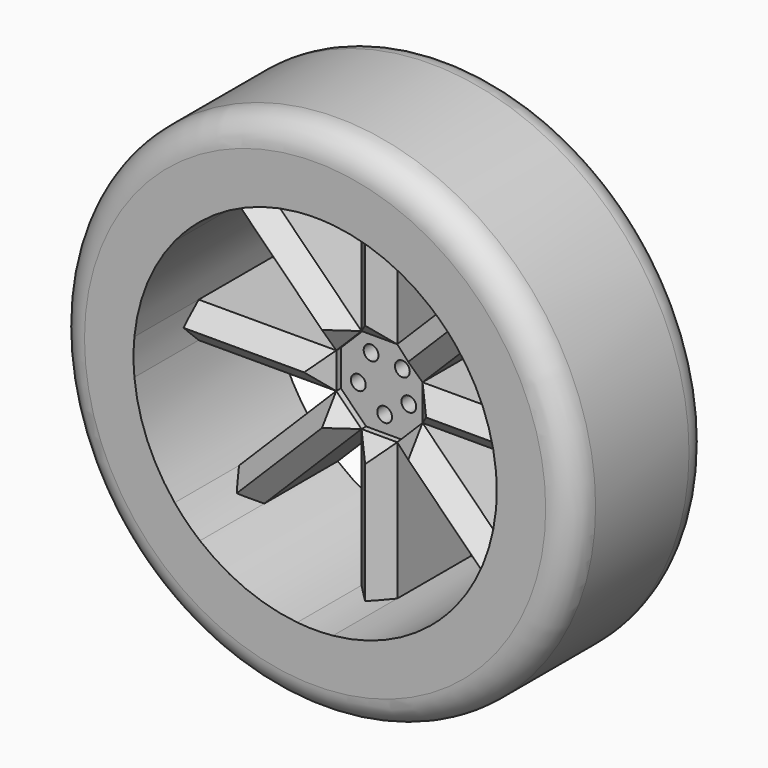
from build123d import *

# Parameters (mm, degrees)
F0_R          = 57.15
F1_DEPTH      = 38.1
F2_DEPTH      = 25.4
F0_R_2        = 1.6372110105
F3_DEPTH      = 19.05
F4_R          = 6.1321024484
F5_SIZE       = 5.08
F5_2_SIZE     = 5.08
F5_3_SIZE     = 5.08
F5_4_SIZE     = 5.08
F5_5_SIZE     = 5.08
F5_6_SIZE     = 5.08
F5_7_SIZE     = 5.08
F5_8_SIZE     = 5.08
F6_T1_DEPTH   = 51.4806015581
F6_2_T1_DEPTH = 51.4806015581
F6_2_T3_DEPTH = 51.4806015581
F6_3_T1_DEPTH = 51.4806015581
F6_4_T1_DEPTH = 51.4806015581
F6_4_T3_DEPTH = 51.4806015581
F6_5_T1_DEPTH = 51.4806015581
F6_6_T1_DEPTH = 51.4806015581
F6_6_T3_DEPTH = 51.4806015581
F6_7_T1_DEPTH = 51.4806015581
F6_8_T1_DEPTH = 51.4806015581
F6_8_T3_DEPTH = 51.4806015581


# Not quite as in the source:
# - a fillet or chamfer that OpenCascade refuses, or shapes differently, is made with other operations: its cross-section is extruded or revolved along the edge and cut away or added


with BuildPart() as f1:
    # F0 (on Front) → F1 (new body)
    with BuildSketch(Plane.XZ):
        Circle(F0_R)
        with BuildLine():
            ThreePointArc((39.9766423626, 3.9533950563), (40.1228666372, 1.979100774), (40.1716475522, 0))
            ThreePointArc((40.1716475522, 0), (40.1228666372, -1.979100774), (39.9766423626, -3.9533950563))
            ThreePointArc((39.9766423626, -3.9533950563), (37.1137629608, -15.3730239691), (31.0632273567, -25.4722824507))
            ThreePointArc((31.0632273567, -25.4722824507), (28.4056443956, -28.4056443956), (25.4722824507, -31.0632273567))
            ThreePointArc((25.4722824507, -31.0632273567), (15.3730239691, -37.1137629608), (3.9533950563, -39.9766423626))
            ThreePointArc((3.9533950563, -39.9766423626), (0, -40.1716475522), (-3.9533950563, -39.9766423626))
            ThreePointArc((-3.9533950563, -39.9766423626), (-15.3730239691, -37.1137629608), (-25.4722824507, -31.0632273567))
            ThreePointArc((-25.4722824507, -31.0632273567), (-28.4056443956, -28.4056443956), (-31.0632273567, -25.4722824507))
            ThreePointArc((-31.0632273567, -25.4722824507), (-37.1137629608, -15.3730239691), (-39.9766423626, -3.9533950563))
            ThreePointArc((-39.9766423626, -3.9533950563), (-40.1716475522, 0), (-39.9766423626, 3.9533950563))
            ThreePointArc((-39.9766423626, 3.9533950563), (-37.1137629608, 15.3730239691), (-31.0632273567, 25.4722824507))
            ThreePointArc((-31.0632273567, 25.4722824507), (-28.4056443956, 28.4056443956), (-25.4722824507, 31.0632273567))
            ThreePointArc((-25.4722824507, 31.0632273567), (-15.3730239691, 37.1137629608), (-3.9533950563, 39.9766423626))
            ThreePointArc((-3.9533950563, 39.9766423626), (0, 40.1716475522), (3.9533950563, 39.9766423626))
            ThreePointArc((3.9533950563, 39.9766423626), (15.3730239691, 37.1137629608), (25.4722824507, 31.0632273567))
            ThreePointArc((25.4722824507, 31.0632273567), (28.4056443956, 28.4056443956), (31.0632273567, 25.4722824507))
            ThreePointArc((31.0632273567, 25.4722824507), (37.1137629608, 15.3730239691), (39.9766423626, 3.9533950563))
        make_face(mode=Mode.SUBTRACT)
    extrude(amount=F1_DEPTH)

    # F4
    f4_edges = [f1.edges().sort_by_distance(p)[0] for p in [
        (-57.15, -38.1, 0),
        (-57.15, 0, 0),
    ]]
    fillet(f4_edges, radius=F4_R)


with BuildPart() as f2:
    # F0 (on Front) → F2 (new body)
    with BuildSketch(Plane.XZ):
        with BuildLine():
            Line((-9.5443399623, -3.9533950563), (-9.5443399623, 3.9533950563))
            Line((-9.5443399623, 3.9533950563), (-39.9766423626, 3.9533950563))
            ThreePointArc((-39.9766423626, 3.9533950563), (-40.1716475522, 0), (-39.9766423626, -3.9533950563))
            Line((-39.9766423626, -3.9533950563), (-9.5443399623, -3.9533950563))
        make_face()
    extrude(amount=F2_DEPTH)

    # F5#4
    f5_4_edges = [f2.edges().sort_by_distance(p)[0] for p in [
        (-9.54434, -25.4, 0),
    ]]
    chamfer(f5_4_edges, length=F5_4_SIZE)

    # F6#3: chamfer of 5.08 on 2 edges, made by hand

    # F6_3_s2 → F6_3_t1 (cut)
    with BuildSketch(Plane.YZ.offset(-53.0407919415)):
        Polygon((-25.4, -1.1266049437), (-20.32, 3.9533950563), (-25.4, 3.9533950563), align=None)
        Polygon((-20.32, -3.9533950563), (-25.4, 1.1266049437), (-25.4, -3.9533950563), align=None)
    extrude(amount=F6_3_T1_DEPTH, mode=Mode.SUBTRACT)


with BuildPart() as f2b:
    # F0 (on Front) → F2, piece 2 (new body)
    with BuildSketch(Plane.XZ):
        with BuildLine():
            Line((-9.5443399623, 3.9533950563), (-3.9533950563, 9.5443399623))
            Line((-3.9533950563, 9.5443399623), (-25.4722824507, 31.0632273567))
            ThreePointArc((-25.4722824507, 31.0632273567), (-28.4056443956, 28.4056443956), (-31.0632273567, 25.4722824507))
            Line((-31.0632273567, 25.4722824507), (-9.5443399623, 3.9533950563))
        make_face()
    extrude(amount=F2_DEPTH)

    # F5#3
    f5_3_edges = [f2b.edges().sort_by_distance(p)[0] for p in [
        (-6.748868, -25.4, 6.748868),
    ]]
    chamfer(f5_3_edges, length=F5_3_SIZE)

    # F6#2: chamfer of 5.08 on 2 edges, made by hand

    # F6_2_s2 → F6_2_t1 (cut)
    with BuildSketch(Plane(origin=(-1.1032212001, 0, 1.1032212001), x_dir=(0, 1, 0), z_dir=(-0.7071067812, 0, 0.7071067812))):
        Polygon((-20.32, -3.9533950563), (-25.4, 1.1266049437), (-25.4, -3.9533950563), align=None)
    extrude(amount=F6_2_T1_DEPTH, mode=Mode.SUBTRACT)

    # F6_2_s4 → F6_2_t3 (cut)
    with BuildSketch(Plane(origin=(-37.5055036613, 0, 37.5055036613), x_dir=(0, 1, 0), z_dir=(0.7071067812, 0, -0.7071067812))):
        Polygon((-25.4, 1.1266049437), (-20.32, -3.9533950563), (-25.4, -3.9533950563), align=None)
    extrude(amount=F6_2_T3_DEPTH, mode=Mode.SUBTRACT)


with BuildPart() as f2c:
    # F0 (on Front) → F2, piece 3 (new body)
    with BuildSketch(Plane.XZ):
        with BuildLine():
            Line((9.5443399623, 3.9533950563), (31.0632273567, 25.4722824507))
            ThreePointArc((31.0632273567, 25.4722824507), (28.4056443956, 28.4056443956), (25.4722824507, 31.0632273567))
            Line((25.4722824507, 31.0632273567), (3.9533950563, 9.5443399623))
            Line((3.9533950563, 9.5443399623), (9.5443399623, 3.9533950563))
        make_face()
    extrude(amount=F2_DEPTH)

    # F5
    f5_edges = [f2c.edges().sort_by_distance(p)[0] for p in [
        (6.748868, -25.4, 6.748868),
    ]]
    chamfer(f5_edges, length=F5_SIZE)

    # F6#8: chamfer of 5.08 on 2 edges, made by hand

    # F6_8_s2 → F6_8_t1 (cut)
    with BuildSketch(Plane(origin=(1.1032212001, 0, 1.1032212001), x_dir=(0, 1, 0), z_dir=(0.7071067812, 0, 0.7071067812))):
        Polygon((-25.4, 1.1266049437), (-20.32, -3.9533950563), (-25.4, -3.9533950563), align=None)
    extrude(amount=F6_8_T1_DEPTH, mode=Mode.SUBTRACT)

    # F6_8_s4 → F6_8_t3 (cut)
    with BuildSketch(Plane(origin=(37.5055036613, 0, 37.5055036613), x_dir=(0, 1, 0), z_dir=(-0.7071067812, 0, -0.7071067812))):
        Polygon((-20.32, -3.9533950563), (-25.4, 1.1266049437), (-25.4, -3.9533950563), align=None)
    extrude(amount=F6_8_T3_DEPTH, mode=Mode.SUBTRACT)


with BuildPart() as f2d:
    # F0 (on Front) → F2, piece 4 (new body)
    with BuildSketch(Plane.XZ):
        with BuildLine():
            Line((-3.9533950563, 9.5443399623), (3.9533950563, 9.5443399623))
            Line((3.9533950563, 9.5443399623), (3.9533950563, 39.9766423626))
            ThreePointArc((3.9533950563, 39.9766423626), (0, 40.1716475522), (-3.9533950563, 39.9766423626))
            Line((-3.9533950563, 39.9766423626), (-3.9533950563, 9.5443399623))
        make_face()
    extrude(amount=F2_DEPTH)

    # F5#2
    f5_2_edges = [f2d.edges().sort_by_distance(p)[0] for p in [
        (0, -25.4, 9.54434),
    ]]
    chamfer(f5_2_edges, length=F5_2_SIZE)

    # F6: chamfer of 5.08 on 2 edges, made by hand

    # F6_s2 → F6_t1 (cut)
    with BuildSketch(Plane.XY.offset(1.5601903834)):
        Polygon((-3.9533950563, -20.32), (1.1266049437, -25.4), (-3.9533950563, -25.4), align=None)
        Polygon((-1.1266049437, -25.4), (3.9533950563, -20.32), (3.9533950563, -25.4), align=None)
    extrude(amount=F6_T1_DEPTH, mode=Mode.SUBTRACT)


with BuildPart() as f2e:
    # F0 (on Front) → F2, piece 5 (new body)
    with BuildSketch(Plane.XZ):
        with BuildLine():
            ThreePointArc((39.9766423626, -3.9533950563), (40.1228666372, -1.979100774), (40.1716475522, 0))
            ThreePointArc((40.1716475522, 0), (40.1228666372, 1.979100774), (39.9766423626, 3.9533950563))
            Line((39.9766423626, 3.9533950563), (9.5443399623, 3.9533950563))
            Line((9.5443399623, 3.9533950563), (9.5443399623, -3.9533950563))
            Line((9.5443399623, -3.9533950563), (39.9766423626, -3.9533950563))
        make_face()
    extrude(amount=F2_DEPTH)

    # F5#8
    f5_8_edges = [f2e.edges().sort_by_distance(p)[0] for p in [
        (9.54434, -25.4, 0),
    ]]
    chamfer(f5_8_edges, length=F5_8_SIZE)

    # F6#7: chamfer of 5.08 on 2 edges, made by hand

    # F6_7_s2 → F6_7_t1 (cut)
    with BuildSketch(Plane.YZ.offset(1.5601903834)):
        Polygon((-20.32, -3.9533950563), (-25.4, 1.1266049437), (-25.4, -3.9533950563), align=None)
        Polygon((-20.32, 3.9533950563), (-25.4, -1.1266049437), (-25.4, 3.9533950563), align=None)
    extrude(amount=F6_7_T1_DEPTH, mode=Mode.SUBTRACT)


with BuildPart() as f2f:
    # F0 (on Front) → F2, piece 6 (new body)
    with BuildSketch(Plane.XZ):
        with BuildLine():
            ThreePointArc((25.4722824507, -31.0632273567), (28.4056443956, -28.4056443956), (31.0632273567, -25.4722824507))
            Line((31.0632273567, -25.4722824507), (9.5443399623, -3.9533950563))
            Line((9.5443399623, -3.9533950563), (3.9533950563, -9.5443399623))
            Line((3.9533950563, -9.5443399623), (25.4722824507, -31.0632273567))
        make_face()
    extrude(amount=F2_DEPTH)

    # F5#7
    f5_7_edges = [f2f.edges().sort_by_distance(p)[0] for p in [
        (6.748868, -25.4, -6.748868),
    ]]
    chamfer(f5_7_edges, length=F5_7_SIZE)

    # F6#6: chamfer of 5.08 on 2 edges, made by hand

    # F6_6_s2 → F6_6_t1 (cut)
    with BuildSketch(Plane(origin=(1.1032212001, 0, -1.1032212001), x_dir=(0, 1, 0), z_dir=(0.7071067812, 0, -0.7071067812))):
        Polygon((-25.4, 1.1266049437), (-20.32, -3.9533950563), (-25.4, -3.9533950563), align=None)
    extrude(amount=F6_6_T1_DEPTH, mode=Mode.SUBTRACT)

    # F6_6_s4 → F6_6_t3 (cut)
    with BuildSketch(Plane(origin=(37.5055036613, 0, -37.5055036613), x_dir=(0, 1, 0), z_dir=(-0.7071067812, 0, 0.7071067812))):
        Polygon((-20.32, -3.9533950563), (-25.4, 1.1266049437), (-25.4, -3.9533950563), align=None)
    extrude(amount=F6_6_T3_DEPTH, mode=Mode.SUBTRACT)


with BuildPart() as f2g:
    # F0 (on Front) → F2, piece 7 (new body)
    with BuildSketch(Plane.XZ):
        with BuildLine():
            Line((3.9533950563, -39.9766423626), (3.9533950563, -9.5443399623))
            Line((3.9533950563, -9.5443399623), (-3.9533950563, -9.5443399623))
            Line((-3.9533950563, -9.5443399623), (-3.9533950563, -39.9766423626))
            ThreePointArc((-3.9533950563, -39.9766423626), (0, -40.1716475522), (3.9533950563, -39.9766423626))
        make_face()
    extrude(amount=F2_DEPTH)

    # F5#6
    f5_6_edges = [f2g.edges().sort_by_distance(p)[0] for p in [
        (0, -25.4, -9.54434),
    ]]
    chamfer(f5_6_edges, length=F5_6_SIZE)

    # F6#5: chamfer of 5.08 on 2 edges, made by hand

    # F6_5_s2 → F6_5_t1 (cut)
    with BuildSketch(Plane.XY.offset(-53.0407919415)):
        Polygon((1.1266049437, -25.4), (-3.9533950563, -20.32), (-3.9533950563, -25.4), align=None)
        Polygon((3.9533950563, -20.32), (-1.1266049437, -25.4), (3.9533950563, -25.4), align=None)
    extrude(amount=F6_5_T1_DEPTH, mode=Mode.SUBTRACT)


with BuildPart() as f2h:
    # F0 (on Front) → F2, piece 8 (new body)
    with BuildSketch(Plane.XZ):
        with BuildLine():
            Line((-25.4722824507, -31.0632273567), (-3.9533950563, -9.5443399623))
            Line((-3.9533950563, -9.5443399623), (-9.5443399623, -3.9533950563))
            Line((-9.5443399623, -3.9533950563), (-31.0632273567, -25.4722824507))
            ThreePointArc((-31.0632273567, -25.4722824507), (-28.4056443956, -28.4056443956), (-25.4722824507, -31.0632273567))
        make_face()
    extrude(amount=F2_DEPTH)

    # F5#5
    f5_5_edges = [f2h.edges().sort_by_distance(p)[0] for p in [
        (-6.748868, -25.4, -6.748868),
    ]]
    chamfer(f5_5_edges, length=F5_5_SIZE)

    # F6#4: chamfer of 5.08 on 2 edges, made by hand

    # F6_4_s2 → F6_4_t1 (cut)
    with BuildSketch(Plane(origin=(-1.1032212001, 0, -1.1032212001), x_dir=(0, 1, 0), z_dir=(-0.7071067812, 0, -0.7071067812))):
        Polygon((-25.4, 1.1266049437), (-20.32, -3.9533950563), (-25.4, -3.9533950563), align=None)
    extrude(amount=F6_4_T1_DEPTH, mode=Mode.SUBTRACT)

    # F6_4_s4 → F6_4_t3 (cut)
    with BuildSketch(Plane(origin=(-37.5055036613, 0, -37.5055036613), x_dir=(0, 1, 0), z_dir=(0.7071067812, 0, 0.7071067812))):
        Polygon((-20.32, -3.9533950563), (-25.4, 1.1266049437), (-25.4, -3.9533950563), align=None)
    extrude(amount=F6_4_T3_DEPTH, mode=Mode.SUBTRACT)


with BuildPart() as f3:
    # F0 (on Front) → F3 (new body)
    with BuildSketch(Plane.XZ):
        Polygon((9.5443399623, -3.9533950563), (9.5443399623, 3.9533950563), (3.9533950563, 9.5443399623), (-3.9533950563, 9.5443399623), (-9.5443399623, 3.9533950563), (-9.5443399623, -3.9533950563), (-3.9533950563, -9.5443399623), (3.9533950563, -9.5443399623), align=None)
        with Locations((-5.6833523544, -1.5429019004)):
            Circle(F0_R_2, mode=Mode.SUBTRACT)
        with Locations((0.1435929958, -5.8873101931)):
            Circle(F0_R_2, mode=Mode.SUBTRACT)
        with Locations((5.4941160495, -2.1203134423)):
            Circle(F0_R_2, mode=Mode.SUBTRACT)
        with Locations((-2.8532490643, 5.1516997229)):
            Circle(F0_R_2, mode=Mode.SUBTRACT)
        with Locations((4.0614213794, 4.2644925416)):
            Circle(F0_R_2, mode=Mode.SUBTRACT)
    extrude(amount=F3_DEPTH)


solid = Compound([f1.part, f2.part, f2b.part, f2c.part, f2d.part, f2e.part, f2f.part, f2g.part, f2h.part, f3.part])
